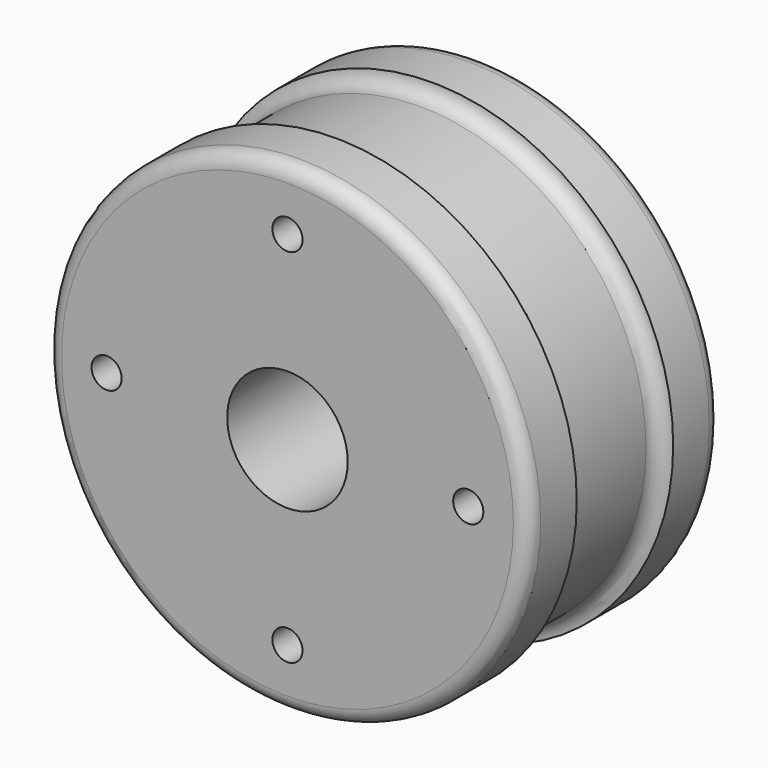
from build123d import *

# Parameters (mm, degrees)
F0_R          = 25.4
F1_DEPTH      = 6.35
F2_R          = 23.8125
F3_DEPTH      = 12.7
F4_R          = 25.4
F5_DEPTH      = 6.35
F6_R          = 6.35
F7_DEPTH      = 25.401
F9_D          = 3.175
F9_DEPTH      = 3.175
F9_TIP        = 0.9538662327
F10_S5_R      = 25.4
F10_T6_DEPTH  = 42
F10_S11_R     = 25.4
F10_T12_DEPTH = 40


# Not quite as in the source:
# - a fillet or chamfer that OpenCascade refuses, or shapes differently, is made with other operations: its cross-section is extruded or revolved along the edge and cut away or added


with BuildPart() as f1:
    # F0 (on Front) → F1 (new body)
    with BuildSketch(Plane.XZ):
        Circle(F0_R)
    extrude(amount=F1_DEPTH)

    # F2 (on face) → F3 (join)
    with BuildSketch(Plane.XZ.offset(6.35)):
        Circle(F2_R)
    extrude(amount=F3_DEPTH)

    # F4 (on face) → F5 (join)
    with BuildSketch(Plane.XZ.offset(19.05)):
        Circle(F4_R)
    extrude(amount=F5_DEPTH)

    # F6 (on face) → F7 (cut, through all)
    with BuildSketch(Plane.XZ.offset(25.4)):
        Circle(F6_R)
    extrude(amount=-F7_DEPTH, mode=Mode.SUBTRACT)

    # F9
    with Locations(Plane.XZ.offset(25.4)):
        with Locations((0, 19.05), (0, -19.05), (-19.05, 0), (19.05, 0)):
            Hole(F9_D / 2, depth=F9_DEPTH)
            with Locations((0, 0, -(F9_DEPTH + F9_TIP / 2))):  # 118° drill point
                Cone(0, F9_D / 2, F9_TIP, mode=Mode.SUBTRACT)

    # F10: fillet of radius 1.6002 on 5 edges, made by hand


with BuildPart() as f10_tool2:
    # F10_s3 → F10_t4 (revolve)
    with BuildSketch(Plane.XY):
        with BuildLine():
            ThreePointArc((23.8125, -7.9502), (24.2811877287, -6.8186877287), (25.4127, -6.35))
            Line((25.4127, -6.35), (23.8125, -6.35))
            Line((23.8125, -6.35), (23.8125, -7.9502))
        make_face()
    revolve(axis=Axis((0, -6.35, 0), (0, -1, 0)))

    # F10_s5 → F10_t6 (intersect, symmetric)
    with BuildSketch(Plane.XZ.offset(7.2)):
        Circle(F10_S5_R)
    extrude(amount=F10_T6_DEPTH, both=True, mode=Mode.INTERSECT)


with BuildPart() as f1_1:
    add(f1.part)

    # F10_t1: union F10_tool2
    add(f10_tool2.part)


with BuildPart() as f10_tool8:
    # F10_s9 → F10_t10 (revolve)
    with BuildSketch(Plane.XY):
        with BuildLine():
            ThreePointArc((25.4127, -19.05), (24.2811877287, -18.5813122713), (23.8125, -17.4498))
            Line((23.8125, -17.4498), (23.8125, -19.05))
            Line((23.8125, -19.05), (25.4127, -19.05))
        make_face()
    revolve(axis=Axis((0, -19.05, 0), (0, -1, 0)))

    # F10_s11 → F10_t12 (intersect, symmetric)
    with BuildSketch(Plane.XZ.offset(17.7)):
        Circle(F10_S11_R)
    extrude(amount=F10_T12_DEPTH, both=True, mode=Mode.INTERSECT)


with BuildPart() as f1_2:
    add(f1_1.part)

    # F10_t7: union F10_tool8
    add(f10_tool8.part)

    # F10_s13 → F10_t14 (revolve, cut)
    with BuildSketch(Plane.XY):
        with BuildLine():
            ThreePointArc((25.4, -23.7998), (24.9313122713, -24.9313122713), (23.7998, -25.4))
            Line((23.7998, -25.4), (25.4, -25.4))
            Line((25.4, -25.4), (25.4, -23.7998))
        make_face()
    revolve(axis=Axis((0, -25.4, 0), (0, -1, 0)), mode=Mode.SUBTRACT)

    # F10_s15 → F10_t16 (revolve, cut)
    with BuildSketch(Plane.XY):
        with BuildLine():
            ThreePointArc((23.7998, 0), (24.9313122713, -0.4686877287), (25.4, -1.6002))
            Line((25.4, -1.6002), (25.4, 0))
            Line((25.4, 0), (23.7998, 0))
        make_face()
    revolve(axis=Axis((0, 0, 0), (0, -1, 0)), mode=Mode.SUBTRACT)


solid = f1_2.part
